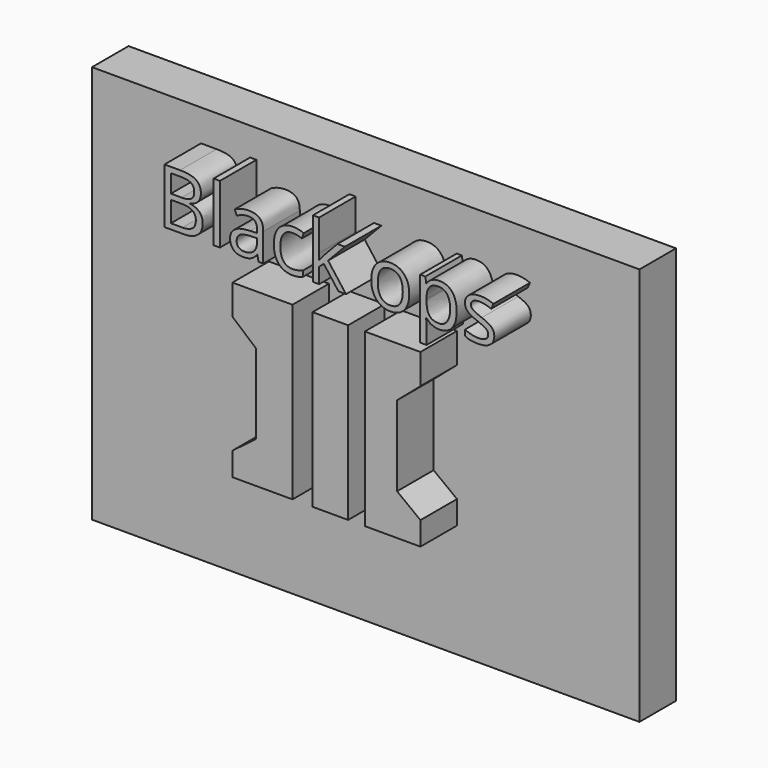
from build123d import *

# Parameters (mm, degrees)
F2_DEPTH     = 25.4
F0_W         = 9.9045271054
F0_H         = 47.665534541
F3_W         = 152.282088995
F3_H         = 110.8068861067
F4_DEPTH     = 12.7
F5_TEXT_SIZE = 21.4941928991
F6_DEPTH     = 25.4


# Not quite as in the source:
# - Text() gives the source's letters only with a copy of the font that has no kerning and outlines rounded to 1/6400 em; it was checked with that copy


with BuildPart() as f2:
    # F0 (on Front) → F2 (new body)
    with BuildSketch(Plane.XZ):
        Polygon((-20.1185699552, -23.3684927225), (-20.1185699552, -11.9163831696), (-26.6184136271, -16.8686453253), (-26.6184136271, -23.3684927225), align=None)
        Polygon((-9.9045261741, 24.2970418185), (-10.5235595256, 24.2970418185), (-20.1185699552, 24.2970418185), (-20.1185699552, 10.3688007221), (-20.1185699552, -11.9163831696), (-20.1185699552, -23.3684927225), (-9.9045261741, -23.3684927225), align=None)
        Polygon((-20.1185699552, 10.3688007221), (-20.1185699552, 24.2970418185), (-26.6184136271, 24.2970418185), (-26.6184136271, 15.9400962293), align=None)
    extrude(amount=F2_DEPTH)



with BuildPart() as f2b:
    # F0 (on Front) → F2, piece 2 (new body)
    with BuildSketch(Plane.XZ):
        with Locations((0.6190333515, 0.464274548)):
            Rectangle(F0_W, F0_H)
    extrude(amount=F2_DEPTH)


with BuildPart() as f2c:
    # F0 (on Front) → F2, piece 3 (new body)
    with BuildSketch(Plane.XZ):
        Polygon((19.1900208592, 24.2970418185), (10.2140419185, 24.2970418185), (10.2140419185, -23.3684927225), (19.1900208592, -23.3684927225), (19.1900208592, -11.9163831696), (19.1900208592, 10.3688007221), align=None)
        Polygon((25.6898645312, 24.2970418185), (19.1900208592, 24.2970418185), (19.1900208592, 10.3688007221), (25.6898645312, 15.9400962293), align=None)
        Polygon((19.1900208592, -11.9163831696), (19.1900208592, -23.3684927225), (25.6898645312, -23.3684927225), (25.6898645312, -16.8686453253), align=None)
    extrude(amount=F2_DEPTH)


with BuildPart() as f2_1:
    add(f2.part)

    add(f2b.part)  # F4 merges F2b

    add(f2c.part)  # F4 merges F2c
    # F3 (on Front) → F4 (join)
    with BuildSketch(Plane.XZ):
        with Locations((0.3095194697, 0.4642736167)):
            Rectangle(F3_W, F3_H)
    extrude(amount=F4_DEPTH)

    # F5 (on Front) → F6 (join)
    with BuildSketch(Plane.XZ):
        with Locations((-47.6163542068, 31.7254345864)):
            Text('Black ops', F5_TEXT_SIZE, font='Open Sans', text_align=(TextAlign.LEFT, TextAlign.BOTTOM))
    extrude(amount=F6_DEPTH)


solid = f2_1.part
